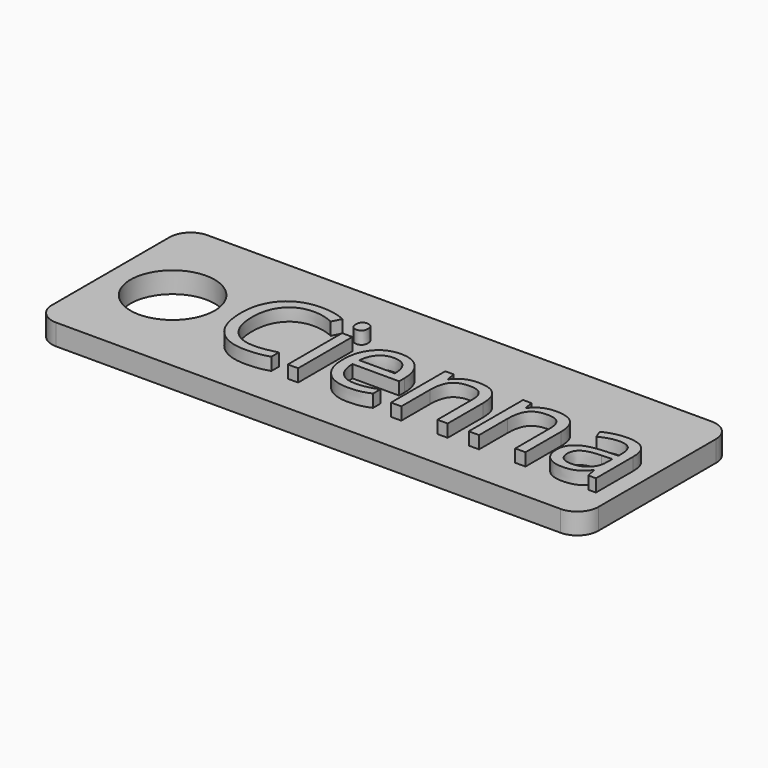
from build123d import *

# Parameters (mm, degrees)
F0_W         = 130
F0_H         = 45
F0_R         = 10
F1_DEPTH     = 5
F2_TEXT_SIZE = 30.1537931793
F3_DEPTH     = 3
F4_R         = 5


# Not quite as in the source:
# - Text() gives the source's letters only with a copy of the font that has no kerning and outlines rounded to 1/6400 em; it was checked with that copy


with BuildPart() as f1:
    # F0 (on Top) → F1 (new body)
    with BuildSketch(Plane.XY):
        with Locations((0.4680925608, 0.3681220487)):
            Rectangle(F0_W, F0_H)
        with Locations((-49.5319074392, 0)):
            Circle(F0_R, mode=Mode.SUBTRACT)
    extrude(amount=F1_DEPTH)

    # F2 (on face) → F3 (join)
    with BuildSketch(Plane.XY.offset(5)):
        with Locations((-33.4138050675, -12.8995459527)):
            Text('Cienna', F2_TEXT_SIZE, font='Open Sans', text_align=(TextAlign.LEFT, TextAlign.BOTTOM))
    extrude(amount=F3_DEPTH)

    # F4
    f4_edges = [f1.edges().sort_by_distance(p)[0] for p in [
        (-64.531907, -22.131878, 2.5),
        (65.468093, -22.131878, 2.5),
        (65.468093, 22.868122, 2.5),
        (-64.531907, 22.868122, 2.5),
    ]]
    fillet(f4_edges, radius=F4_R)


solid = f1.part
